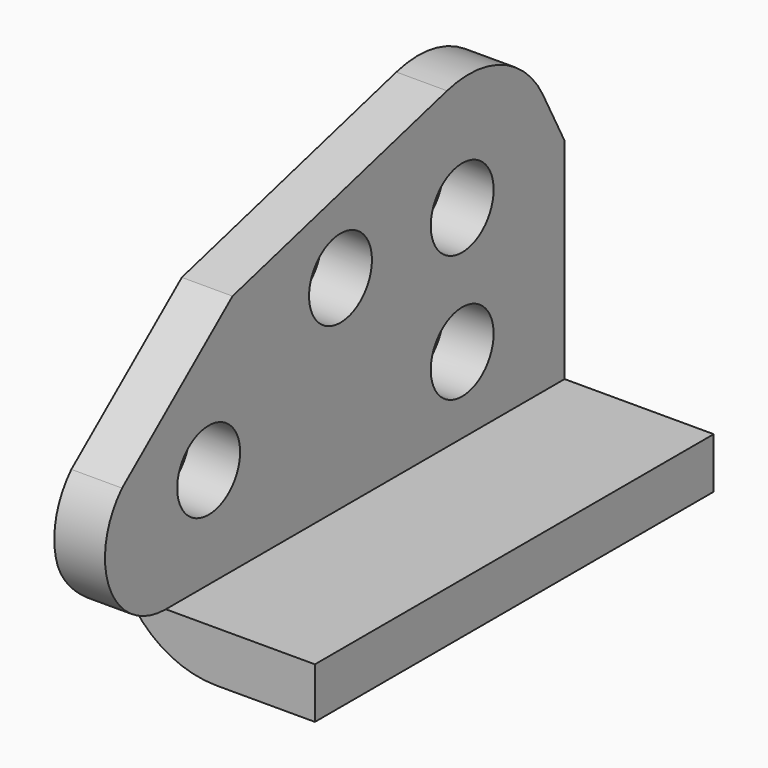
from build123d import *

# Parameters (mm, degrees)
F0_R        = 1.55
F1_DEPTH    = 2
F2_W        = 5.8800544143
F2_H        = 19.6606332908
F2_W_2      = 2
F3_DEPTH    = 2
F4_T1_DEPTH = 39.6606332908


# Not quite as in the source:
# - a fillet or chamfer that OpenCascade refuses, or shapes differently, is made with other operations: its cross-section is extruded or revolved along the edge and cut away or added


with BuildPart() as f1:
    # F0 (on Right) → F1 (new body)
    with BuildSketch(Plane.YZ):
        with BuildLine():
            Line((-14.6106332908, -3), (-13.2183143869, -3))
            Line((-13.2183143869, -3), (5.05, -3))
            Line((5.05, -3), (5.05, 5.273589902))
            Line((5.05, 5.273589902), (3.9867715302, 7.2948440555))
            ThreePointArc((3.9867715302, 7.2948440555), (1.9828252763, 9.159944049), (-0.7469684056, 9.3664023457))
            Line((-0.7469684056, 9.3664023457), (-11.3228132649, 6.5356446488))
            Line((-11.3228132649, 6.5356446488), (-16.7690545021, 2.0835589443))
            ThreePointArc((-16.7690545021, 2.0835589443), (-17.372034822, -1.1724596298), (-14.6106332908, -3))
        make_face()
        with Locations((-12.5, 0.9715808555)):
            Circle(F0_R, mode=Mode.SUBTRACT)
        Circle(F0_R, mode=Mode.SUBTRACT)
        with Locations((-6, 5)):
            Circle(F0_R, mode=Mode.SUBTRACT)
        with Locations((0, 5)):
            Circle(F0_R, mode=Mode.SUBTRACT)
    extrude(amount=F1_DEPTH)

    # F2 (on face) → F3 (join)
    with BuildSketch(Plane(origin=(0, 0, -3), x_dir=(1, 0, 0), z_dir=(0, 0, -1))):
        with Locations((4.9400272071, 4.7803166454)):
            Rectangle(F2_W, F2_H)
        with Locations((1, 4.7803166454)):
            Rectangle(F2_W_2, F2_H)
    extrude(amount=F3_DEPTH)

    # F4: fillet of radius 4 on 1 edges, made by hand

    # F4_s2 → F4_t1 (cut)
    with BuildSketch(Plane.XZ.offset(-15.05)):
        with BuildLine():
            ThreePointArc((4, -5), (1.1715728753, -3.8284271247), (0, -1))
            Line((0, -1), (0, -5))
            Line((0, -5), (4, -5))
        make_face()
    extrude(amount=F4_T1_DEPTH, mode=Mode.SUBTRACT)


solid = f1.part
